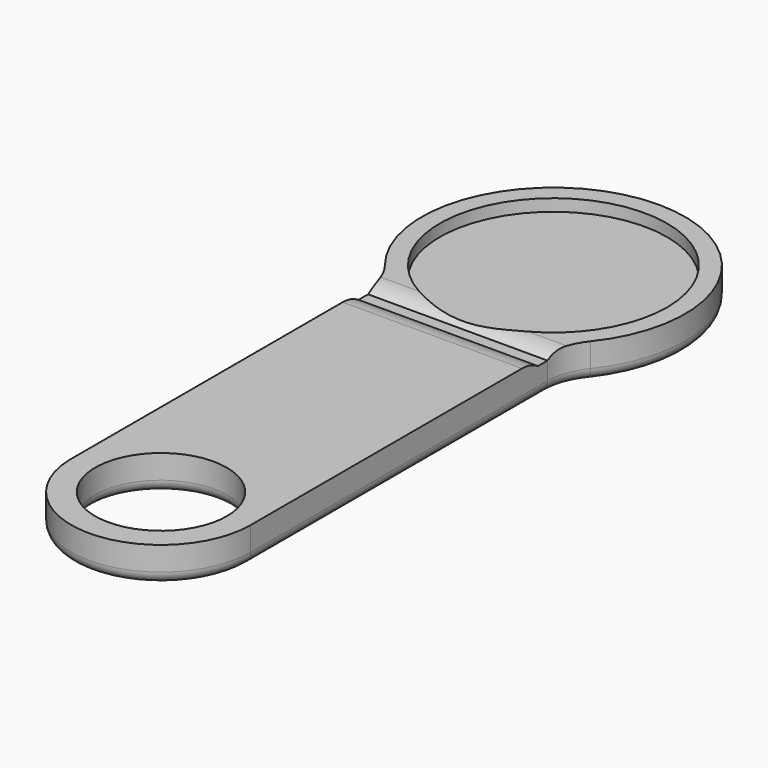
from build123d import *

# Parameters (mm, degrees)
F1_DEPTH    = 3
F2_R        = 9.5
F3_DEPTH    = 1
F4_W        = 14.9929515668
F4_H        = 1
F5_DEPTH    = 0.5
F6_T1_DEPTH = 23.2845135427
F7_R        = 5.5
F8_DEPTH    = 3.0010001
F9_F1_R     = 1


# Not quite as in the source:
# - a fillet or chamfer that OpenCascade refuses, or shapes differently, is made with other operations: its cross-section is extruded or revolved along the edge and cut away or added


with BuildPart() as f1:
    # F0 (on Top) → F1 (new body)
    with BuildSketch(Plane.XY):
        with BuildLine():
            ThreePointArc((7.5, -9.9874921777), (7.781353478, -8.3338976083), (8.59375, -6.8664008722))
            ThreePointArc((8.59375, -6.8664008722), (-0.0038797807, 10.9999993158), (-8.5889042022, -6.8724613208))
            ThreePointArc((-8.5889042022, -6.8724613208), (-7.7748885732, -8.3410486079), (-7.4929515668, -9.9963073757))
            Line((-7.4929515668, -9.9963073757), (-7.4929515668, -40.6749202897))
            Line((-7.4929515668, -40.6749202897), (-7.4929515668, -41.3250797103))
            ThreePointArc((-7.4929515668, -41.3250797103), (0.162578057, -48.4982376846), (7.5, -41))
            Line((7.5, -41), (7.5, -9.9874921777))
        make_face()
    extrude(amount=F1_DEPTH)

    # F2 (on face) → F3 (cut)
    with BuildSketch(Plane.XY.offset(3)):
        Circle(F2_R)
    extrude(amount=-F3_DEPTH, mode=Mode.SUBTRACT)

    # F4 (on face) → F5 (cut)
    with BuildSketch(Plane.XY.offset(3)):
        with Locations((0.0035242166, -10.5)):
            Rectangle(F4_W, F4_H)
    extrude(amount=-F5_DEPTH, mode=Mode.SUBTRACT)

    # F6: fillet of radius 3 on 2 edges, made by hand

    # F6_s2 → F6_t1 (cut)
    with BuildSketch(Plane.YZ.offset(-11.6387325547)):
        with BuildLine():
            ThreePointArc((-12.6583123952, 3), (-11.7922869914, 2.8722813233), (-11, 2.5))
            Line((-11, 2.5), (-11, 3))
            Line((-11, 3), (-12.6583123952, 3))
        make_face()
        with BuildLine():
            ThreePointArc((-8.3416876048, 3), (-9.2077130086, 2.8722813233), (-10, 2.5))
            Line((-10, 2.5), (-10, 3))
            Line((-10, 3), (-8.3416876048, 3))
        make_face()
    extrude(amount=F6_T1_DEPTH, mode=Mode.SUBTRACT)

    # F7 (on face) → F8 (cut, through all)
    with BuildSketch(Plane.XY.offset(3)):
        with Locations((0, -41)):
            Circle(F7_R)
    extrude(amount=-F8_DEPTH, mode=Mode.SUBTRACT)

    # F9: fillet of radius 1 on 7 edges, made by hand

    # F9_f1
    f9_f1_edges = [f1.edges().sort_by_distance(p)[0] for p in [
        (-7.7748885732, -8.3410486079, 0),
        (-0.0038797807, 10.9999993158, 0),
        (-7.4929515668, -25.660693543, 0),
        (7.781353478, -8.3338976083, 0),
        (0.162578057, -48.4982376846, 0),
        (7.5, -25.4937460889, 0),
    ]]
    fillet(f9_f1_edges, radius=F9_F1_R)

    # F9_s2 → F9_t3 (revolve, cut)
    with BuildSketch(Plane.XZ.offset(41)):
        with BuildLine():
            ThreePointArc((6.5, 0), (5.7928932188, 0.2928932188), (5.5, 1))
            Line((5.5, 1), (5.48, 1))
            Line((5.48, 1), (5.48, -0.02))
            Line((5.48, -0.02), (6.5, -0.02))
            Line((6.5, -0.02), (6.5, 0))
        make_face()
    revolve(axis=Axis((0, -41, 0), (0, 0, 1)), mode=Mode.SUBTRACT)


solid = f1.part
